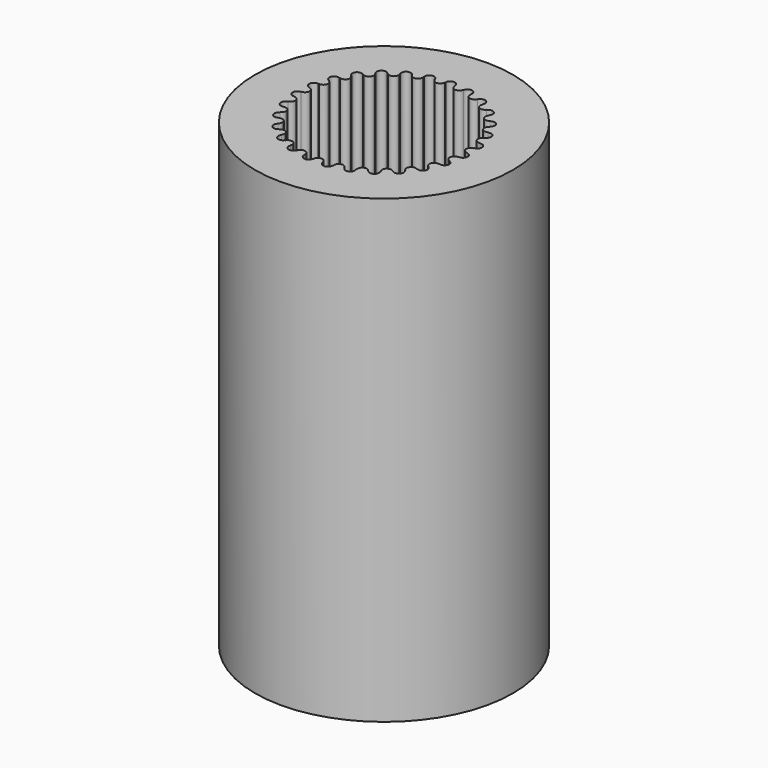
from build123d import *

# Parameters (mm, degrees)
F0_R     = 7
F1_DEPTH = 25


with BuildPart() as f1:
    # F0 (on Top) → F1 (new body)
    with BuildSketch(Plane.XY):
        Circle(F0_R)
        with BuildLine():
            ThreePointArc((4.4999467421, 0.0218933428), (4.4999866855, 0.0109467038), (4.5, 0))
            ThreePointArc((4.5, 0), (4.499999901, -0.0009440021), (4.4999996039, -0.0018880042))
            ThreePointArc((4.4999996039, -0.0018880042), (4.6722019825, -0.0775220264), (4.7429503115, -0.2517885994))
            ThreePointArc((4.7429503115, -0.2517885994), (4.6621704259, -0.4358118394), (4.4720338884, -0.5009120693))
            ThreePointArc((4.4720338884, -0.5009120693), (4.4706946769, -0.5127271263), (4.4693242502, -0.5245386035))
            ThreePointArc((4.4693242502, -0.5245386035), (4.6223829499, -0.6083851155), (4.6832973562, -0.7719291104))
            ThreePointArc((4.6832973562, -0.7719291104), (4.5915258656, -0.9654846291), (4.3835874457, -1.01693712))
            ThreePointArc((4.3835874457, -1.01693712), (4.3808850095, -1.0285166667), (4.3781519852, -1.040089032))
            ThreePointArc((4.3781519852, -1.040089032), (4.5119142579, -1.1293532515), (4.5636351508, -1.2816207651))
            ThreePointArc((4.5636351508, -1.2816207651), (4.460336155, -1.484053014), (4.2358046277, -1.5191968785))
            ThreePointArc((4.2358046277, -1.5191968785), (4.2317755471, -1.5303841736), (4.2277169195, -1.5415607832))
            ThreePointArc((4.2277169195, -1.5415607832), (4.3423845204, -1.6334890402), (4.3855834466, -1.7739643615))
            ThreePointArc((4.3855834466, -1.7739643615), (4.2702600875, -1.9845877277), (4.0306858273, -2.0008927411))
            ThreePointArc((4.0306858273, -2.0008927411), (4.0253846401, -2.011536353), (4.0200553469, -2.02216592))
            ThreePointArc((4.0200553469, -2.02216592), (4.116174988, -2.1140881649), (4.151552357, -2.2422955214))
            ThreePointArc((4.151552357, -2.2422955214), (4.0237485016, -2.4603966499), (3.7710075389, -2.4555044576))
            ThreePointArc((3.7710075389, -2.4555044576), (3.764506002, -2.4654603141), (3.7579781807, -2.4753989564))
            ThreePointArc((3.7579781807, -2.4753989564), (3.8364270221, -2.5647697304), (3.864709734, -2.6802748998))
            ThreePointArc((3.864709734, -2.6802748998), (3.7240115191, -2.9051151092), (3.4602847759, -2.8768783898))
            ThreePointArc((3.4602847759, -2.8768783898), (3.4526708943, -2.8860117282), (3.4450329057, -2.8951249159))
            ThreePointArc((3.4450329057, -2.8951249159), (3.5069993046, -2.9795622136), (3.5289382883, -3.0819739943))
            ThreePointArc((3.5289382883, -3.0819739943), (3.3749755225, -3.3127917788), (3.102723491, -3.2593108072))
            ThreePointArc((3.102723491, -3.2593108072), (3.0941003266, -3.2674979983), (3.0854555587, -3.2756623751))
            ThreePointArc((3.0854555587, -3.2756623751), (3.1324153628, -3.3529838574), (3.1487830325, -3.4419553935))
            ThreePointArc((3.1487830325, -3.4419553935), (2.9812304495, -3.677969002), (2.7031636451, -3.5976250927))
            ThreePointArc((2.7031636451, -3.5976250927), (2.6936479212, -3.6047553144), (2.6841133898, -3.611860367))
            ThreePointArc((2.6841133898, -3.611860367), (2.7178021206, -3.6801164221), (2.7293897599, -3.755346378))
            ThreePointArc((2.7293897599, -3.755346378), (2.5479681207, -3.9957564618), (2.2670136924, -3.8872418137))
            ThreePointArc((2.2670136924, -3.8872418137), (2.2567342142, -3.8932185511), (2.2464389791, -3.8991681053))
            ThreePointArc((2.2464389791, -3.8991681053), (2.268820309, -3.9566712966), (2.2764353908, -4.0179048778))
            ThreePointArc((2.2764353908, -4.0179048778), (2.080912429, -4.261897198), (1.8001773723, -4.1242407093))
            ThreePointArc((1.8001773723, -4.1242407093), (1.7892732831, -4.128983061), (1.7783567009, -4.1336965835))
            ThreePointArc((1.7783567009, -4.1336965835), (1.7915876777, -4.1790470769), (1.7960511297, -4.2260768929))
            ThreePointArc((1.7960511297, -4.2260768929), (1.5862423383, -4.4728250778), (1.3089737957, -4.3054137551))
            ThreePointArc((1.3089737957, -4.3054137551), (1.2975926935, -4.3088575286), (1.2862025314, -4.3122712169))
            ThreePointArc((1.2862025314, -4.3122712169), (1.2925960487, -4.3443778338), (1.2947394726, -4.3770446005))
            ThreePointArc((1.2947394726, -4.3770446005), (1.070508729, -4.6257129447), (0.8000519092, -4.4283085871))
            ThreePointArc((0.8000519092, -4.4283085871), (0.7883478491, -4.4304071674), (0.7766382847, -4.4324748138))
            ThreePointArc((0.7766382847, -4.4324748138), (0.7786233347, -4.4505714179), (0.7792861897, -4.468764497))
            ThreePointArc((0.7792861897, -4.468764497), (0.5405462167, -4.7185107918), (0.2803004953, -4.4912616972))
            ThreePointArc((0.2803004953, -4.4912616972), (0.2684319038, -4.4919866777), (0.2565614381, -4.4926802945))
            ThreePointArc((0.2565614381, -4.4926802945), (0.2566417125, -4.4963372852), (0.2566684725, -4.499995059))
            ThreePointArc((0.2566684725, -4.499995059), (0.0033811338, -4.7499734449), (-0.2432450747, -4.49342095))
            ThreePointArc((-0.2432450747, -4.49342095), (-0.255117544, -4.4927625175), (-0.2669882321, -4.4920727158))
            ThreePointArc((-0.2669882321, -4.4920727158), (-0.5447083709, -4.7186643015), (-0.7634980719, -4.4347571178))
            ThreePointArc((-0.7634980719, -4.4347571178), (-0.7752137129, -4.4327241849), (-0.7869239413, -4.4306603019))
            ThreePointArc((-0.7869239413, -4.4306603019), (-1.0890824956, -4.6234618326), (-1.2734163355, -4.3160642762))
            ThreePointArc((-1.2734163355, -4.3160642762), (-1.284816565, -4.3126843606), (-1.2962078237, -4.3092743331))
            ThreePointArc((-1.2962078237, -4.3092743331), (-1.618714766, -4.4656760413), (-1.7660975963, -4.1389490551))
            ThreePointArc((-1.7660975963, -4.1389490551), (-1.7770281003, -4.1342679075), (-1.7879461969, -4.1295578937))
            ThreePointArc((-1.7879461969, -4.1295578937), (-2.1264360633, -4.2474427211), (-2.2348729054, -3.9058088915))
            ThreePointArc((-2.2348729054, -3.9058088915), (-2.2451857283, -3.899889876), (-2.255482875, -3.8939436309))
            ThreePointArc((-2.255482875, -3.8939436309), (-2.6053738563, -3.9717158847), (-2.6733969057, -3.619799578))
            ThreePointArc((-2.6733969057, -3.619799578), (-2.6829524529, -3.6127228147), (-2.6924892672, -3.6056208267))
            ThreePointArc((-2.6924892672, -3.6056208267), (-3.0490452281, -3.6422277794), (-3.0757337228, -3.2847925454))
            ThreePointArc((-3.0757337228, -3.2847925454), (-3.0844026501, -3.2766538255), (-3.0930500415, -3.2684922274))
            ThreePointArc((-3.0930500415, -3.2684922274), (-3.4514446295, -3.2634383661), (-3.4364373131, -2.9053224594))
            ThreePointArc((-3.4364373131, -2.9053224594), (-3.4441022776, -2.8962319489), (-3.4517431947, -2.8871212163))
            ThreePointArc((-3.4517431947, -2.8871212163), (-3.8071251696, -2.8404749503), (-3.7506251817, -2.4865258387))
            ThreePointArc((-3.7506251817, -2.4865258387), (-3.7571824301, -2.476606587), (-3.7637134453, -2.4666700432))
            ThreePointArc((-3.7637134453, -2.4666700432), (-4.1112723457, -2.3790627776), (-4.0140444718, -2.0340715273))
            ThreePointArc((-4.0140444718, -2.0340715273), (-4.0194052451, -2.0234578017), (-4.0247379543, -2.012829948))
            ThreePointArc((-4.0247379543, -2.012829948), (-4.3597692121, -1.8854475376), (-4.2231295318, -1.5540839609))
            ThreePointArc((-4.2231295318, -1.5540839609), (-4.2272212664, -1.5429194291), (-4.2312834858, -1.5317441244))
            ThreePointArc((-4.2312834858, -1.5317441244), (-4.5492521077, -1.3663108214), (-4.3750501799, -1.0530602659))
            ThreePointArc((-4.3750501799, -1.0530602659), (-4.3778174899, -1.0414960514), (-4.3805542332, -1.029924565))
            ThreePointArc((-4.3805542332, -1.029924565), (-4.677156186, -0.8286796797), (-4.4677500134, -0.5377823145))
            ThreePointArc((-4.4677500134, -0.5377823145), (-4.4691554405, -0.5259749509), (-4.4705296631, -0.5141639148))
            ThreePointArc((-4.4705296631, -0.5141639148), (-4.7417501336, -0.2798315043), (-4.4999742446, -0.0152249251))
            ThreePointArc((-4.4999742446, -0.0152249251), (-4.4999987648, -0.0033342372), (-4.4999918652, 0.0085564741))
            ThreePointArc((-4.4999918652, 0.0085564741), (-4.7421596047, 0.2728044791), (-4.4712866852, 0.5075385493))
            ThreePointArc((-4.4712866852, 0.5075385493), (-4.4699299666, 0.5193516089), (-4.4685420382, 0.5311610422))
            ThreePointArc((-4.4685420382, 0.5311610422), (-4.6783790567, 0.8217477726), (-4.3820756509, 1.0234319662))
            ThreePointArc((-4.3820756509, 1.0234319662), (-4.3793560582, 1.0350074955), (-4.376605888, 1.0465757981))
            ThreePointArc((-4.376605888, 1.0465757981), (-4.5512718251, 1.3595678629), (-4.2335487052, 1.5254721764))
            ThreePointArc((-4.2335487052, 1.5254721764), (-4.2295030507, 1.5366534886), (-4.2254278651, 1.5478240716))
            ThreePointArc((-4.2254278651, 1.5478240716), (-4.3625584374, 1.8789848005), (-4.0277163132, 2.0068635481))
            ThreePointArc((-4.0277163132, 2.0068635481), (-4.0223993592, 2.0174992926), (-4.01705432, 2.0281209505))
            ThreePointArc((-4.01705432, 2.0281209505), (-4.1147933237, 2.3729677417), (-3.7673646286, 2.4610899526))
            ThreePointArc((-3.7673646286, 2.4610899526), (-3.7608483455, 2.4710361637), (-3.7543058034, 2.4809651216))
            ThreePointArc((-3.7543058034, 2.4809651216), (-3.8113302403, 2.8348301182), (-3.4560177799, 2.8820029675))
            ThreePointArc((-3.4560177799, 2.8820029675), (-3.4483903723, 2.891125013), (-3.4407388873, 2.9002268721))
            ThreePointArc((-3.4407388873, 2.9002268721), (-3.456276873, 3.2583201465), (-3.0978901677, 3.2639051011))
            ThreePointArc((-3.0978901677, 3.2639051011), (-3.0892548803, 3.2720795046), (-3.0805980232, 3.2802310619))
            ThreePointArc((-3.0805980232, 3.2802310619), (-3.054439235, 3.6377054526), (-2.6978294184, 3.6016269142))
            ThreePointArc((-2.6978294184, 3.6016269142), (-2.6883031388, 3.6087430269), (-2.678758089, 3.6158339426))
            ThreePointArc((-2.678758089, 3.6158339426), (-2.611256613, 3.9678506652), (-2.2612507666, 3.8905969941))
            ThreePointArc((-2.2612507666, 3.8905969941), (-2.2509624428, 3.8965584919), (-2.2406584025, 3.9024927833))
            ThreePointArc((-2.2406584025, 3.9024927833), (-2.1327279408, 4.2442869284), (-1.7940637545, 4.1269038328))
            ThreePointArc((-1.7940637545, 4.1269038328), (-1.7831526496, 4.1316300207), (-1.7722290945, 4.1363273609))
            ThreePointArc((-1.7722290945, 4.1363273609), (-1.6253305972, 4.4632723925), (-1.3025922399, 4.3073487735))
            ThreePointArc((-1.3025922399, 4.3073487735), (-1.291206047, 4.3107756778), (-1.2798108387, 4.3141724835))
            ThreePointArc((-1.2798108387, 4.3141724835), (-1.0959327283, 4.6218428635), (-0.7934887965, 4.429489308))
            ThreePointArc((-0.7934887965, 4.429489308), (-0.7817816394, 4.431570542), (-0.7700690238, 4.4336208339))
            ThreePointArc((-0.7700690238, 4.4336208339), (-0.5517002802, 4.7178519265), (-0.2736446642, 4.4916721383))
            ThreePointArc((-0.2736446642, 4.4916721383), (-0.2617750113, 4.4923795302), (-0.2499035308, 4.4930555556))
            ThreePointArc((-0.2499035308, 4.4930555556), (-0.0034725572, 4.7499758815), (0.25, 4.5))
            ThreePointArc((0.25, 4.5), (0.2499758815, 4.4965274428), (0.2499035308, 4.4930555556))
            ThreePointArc((0.2499035308, 4.4930555556), (0.255117544, 4.4927625175), (0.2603312137, 4.4924634288))
            ThreePointArc((0.2603312137, 4.4924634288), (0.5201193193, 4.7208440575), (0.759414462, 4.4710733505))
            ThreePointArc((0.759414462, 4.4710733505), (0.758791431, 4.4534345488), (0.7569254433, 4.4358836632))
            ThreePointArc((0.7569254433, 4.4358836632), (0.7686440841, 4.4338680937), (0.780357358, 4.4318215661))
            ThreePointArc((0.780357358, 4.4318215661), (1.0504868514, 4.6303708881), (1.2752704044, 4.3816458777))
            ThreePointArc((1.2752704044, 4.3816458777), (1.2731989807, 4.3495301331), (1.267019036, 4.317946591))
            ThreePointArc((1.267019036, 4.317946591), (1.2784242616, 4.3145835729), (1.289820561, 4.3111904296))
            ThreePointArc((1.289820561, 4.3111904296), (1.5668908867, 4.4797452241), (1.777248255, 4.2329083108))
            ThreePointArc((1.777248255, 4.2329083108), (1.7728887354, 4.1864243953), (1.7599622198, 4.1415616602))
            ThreePointArc((1.7599622198, 4.1415616602), (1.7708996487, 4.1368967154), (1.781824713, 4.1322028861))
            ThreePointArc((1.781824713, 4.1322028861), (2.0624877777, 4.2709867763), (2.2585532259, 4.0268739661))
            ThreePointArc((2.2585532259, 4.0268739661), (2.2510736567, 3.966179315), (2.2290825005, 3.9091164226))
            ThreePointArc((2.2290825005, 3.9091164226), (2.2394040835, 3.9032126961), (2.2497100305, 3.8972817166))
            ThreePointArc((2.2497100305, 3.8972817166), (2.5307141606, 4.0068936583), (2.7126703583, 3.7663317308))
            ThreePointArc((2.7126703583, 3.7663317308), (2.7012493529, 3.6916319093), (2.6680298516, 3.6237572643))
            ThreePointArc((2.6680298516, 3.6237572643), (2.6775958753, 3.616694669), (2.6871432035, 3.6096068212))
            ThreePointArc((2.6871432035, 3.6096068212), (2.9653753054, 3.6910046043), (3.1334527085, 3.4548083127))
            ThreePointArc((3.1334527085, 3.4548083127), (3.1172822297, 3.3663563198), (3.0708626682, 3.2893468156))
            ThreePointArc((3.0708626682, 3.2893468156), (3.0795436465, 3.281220951), (3.088203123, 3.2730721763))
            ThreePointArc((3.088203123, 3.2730721763), (3.3607284835, 3.3275511906), (3.5152045537, 3.0965205025))
            ThreePointArc((3.5152045537, 3.0965205025), (3.4934926499, 2.9946159141), (3.4321281926, 2.9104116667))
            ThreePointArc((3.4321281926, 2.9104116667), (3.4398066197, 2.9013325247), (3.4474610295, 2.8922331251))
            ThreePointArc((3.4474610295, 2.8922331251), (3.7115602241, 2.9214007075), (3.8527584891, 2.696318095))
            ThreePointArc((3.8527584891, 2.696318095), (3.824731977, 2.5813060492), (3.7469363237, 2.4920810954))
            ThreePointArc((3.7469363237, 2.4920810954), (3.7535082641, 2.4821715717), (3.7600539969, 2.472244717))
            ThreePointArc((3.7600539969, 2.472244717), (4.0132564165, 2.4779904525), (4.1415453741, 2.2596182423))
            ThreePointArc((4.1415453741, 2.2596182423), (4.1064524572, 2.1318882707), (4.0110258089, 2.0400176373))
            ThreePointArc((4.0110258089, 2.0400176373), (4.0164023046, 2.0294118674), (4.0217507571, 2.0187919278))
            ThreePointArc((4.0217507571, 2.0187919278), (4.2618643103, 2.0032543356), (4.3776561806, 1.7923321273))
            ThreePointArc((4.3776561806, 1.7923321273), (4.3347689953, 1.6523168353), (4.2208219246, 1.5603404375))
            ThreePointArc((4.2208219246, 1.5603404375), (4.2249301992, 1.5491819814), (4.2290089747, 1.5380127087))
            ThreePointArc((4.2290089747, 1.5380127087), (4.454145576, 1.5035427883), (4.5578949054, 1.3007849491))
            ThreePointArc((4.5578949054, 1.3007849491), (4.5065119864, 1.1489585511), (4.3734848642, 1.0595424212))
            ThreePointArc((4.3734848642, 1.0595424212), (4.376269308, 1.0479823202), (4.379023196, 1.036414902))
            ThreePointArc((4.379023196, 1.036414902), (4.5876197103, 0.9855370602), (4.6798218315, 0.7916303057))
            ThreePointArc((4.6798218315, 0.7916303057), (4.6192704875, 0.6285070187), (4.4669481775, 0.5444024059))
            ThreePointArc((4.4669481775, 0.5444024059), (4.4683711002, 0.5325971379), (4.4697628239, 0.5207881512))
            ThreePointArc((4.4697628239, 0.5207881512), (4.6605971976, 0.4561590617), (4.7417865523, 0.2717601299))
            ThreePointArc((4.7417865523, 0.2717601299), (4.6714251443, 0.0978924323), (4.4999467421, 0.0218933428))
        make_face(mode=Mode.SUBTRACT)
        with BuildLine():
            ThreePointArc((4.4697628239, 0.5207881512), (4.4917865523, 0.2717601299), (4.4999467421, 0.0218933428))
            ThreePointArc((4.4999467421, 0.0218933428), (4.6714251443, 0.0978924323), (4.7417865523, 0.2717601299))
            ThreePointArc((4.7417865523, 0.2717601299), (4.6605971976, 0.4561590617), (4.4697628239, 0.5207881512))
        make_face()
        with BuildLine():
            ThreePointArc((4.6832973562, -0.7719291104), (4.6223829499, -0.6083851155), (4.4693242502, -0.5245386035))
            ThreePointArc((4.4693242502, -0.5245386035), (4.4332973562, -0.7719291104), (4.3835874457, -1.01693712))
            ThreePointArc((4.3835874457, -1.01693712), (4.5915258656, -0.9654846291), (4.6832973562, -0.7719291104))
        make_face()
        with BuildLine():
            ThreePointArc((4.2290089747, 1.5380127087), (4.3078949054, 1.3007849491), (4.3734848642, 1.0595424212))
            ThreePointArc((4.3734848642, 1.0595424212), (4.5065119864, 1.1489585511), (4.5578949054, 1.3007849491))
            ThreePointArc((4.5578949054, 1.3007849491), (4.454145576, 1.5035427883), (4.2290089747, 1.5380127087))
        make_face()
        with BuildLine():
            ThreePointArc((4.3855834466, -1.7739643615), (4.3423845204, -1.6334890402), (4.2277169195, -1.5415607832))
            ThreePointArc((4.2277169195, -1.5415607832), (4.1355834466, -1.7739643615), (4.0306858273, -2.0008927411))
            ThreePointArc((4.0306858273, -2.0008927411), (4.2702600875, -1.9845877277), (4.3855834466, -1.7739643615))
        make_face()
        with BuildLine():
            ThreePointArc((3.7600539969, 2.472244717), (3.8915453741, 2.2596182423), (4.0110258089, 2.0400176373))
            ThreePointArc((4.0110258089, 2.0400176373), (4.1064524572, 2.1318882707), (4.1415453741, 2.2596182423))
            ThreePointArc((4.1415453741, 2.2596182423), (4.0132564165, 2.4779904525), (3.7600539969, 2.472244717))
        make_face()
        with BuildLine():
            ThreePointArc((3.864709734, -2.6802748998), (3.8364270221, -2.5647697304), (3.7579781807, -2.4753989564))
            ThreePointArc((3.7579781807, -2.4753989564), (3.614709734, -2.6802748998), (3.4602847759, -2.8768783898))
            ThreePointArc((3.4602847759, -2.8768783898), (3.7240115191, -2.9051151092), (3.864709734, -2.6802748998))
        make_face()
        with BuildLine():
            ThreePointArc((3.088203123, 3.2730721763), (3.2652045537, 3.0965205025), (3.4321281926, 2.9104116667))
            ThreePointArc((3.4321281926, 2.9104116667), (3.4934926499, 2.9946159141), (3.5152045537, 3.0965205025))
            ThreePointArc((3.5152045537, 3.0965205025), (3.3607284835, 3.3275511906), (3.088203123, 3.2730721763))
        make_face()
        with BuildLine():
            ThreePointArc((3.1487830325, -3.4419553935), (3.1324153628, -3.3529838574), (3.0854555587, -3.2756623751))
            ThreePointArc((3.0854555587, -3.2756623751), (2.8987830325, -3.4419553935), (2.7031636451, -3.5976250927))
            ThreePointArc((2.7031636451, -3.5976250927), (2.9812304495, -3.677969002), (3.1487830325, -3.4419553935))
        make_face()
        with BuildLine():
            ThreePointArc((2.2497100305, 3.8972817166), (2.4626703583, 3.7663317308), (2.6680298516, 3.6237572643))
            ThreePointArc((2.6680298516, 3.6237572643), (2.7012493529, 3.6916319093), (2.7126703583, 3.7663317308))
            ThreePointArc((2.7126703583, 3.7663317308), (2.5307141606, 4.0068936583), (2.2497100305, 3.8972817166))
        make_face()
        with BuildLine():
            ThreePointArc((2.2764353908, -4.0179048778), (2.268820309, -3.9566712966), (2.2464389791, -3.8991681053))
            ThreePointArc((2.2464389791, -3.8991681053), (2.0264353908, -4.0179048778), (1.8001773723, -4.1242407093))
            ThreePointArc((1.8001773723, -4.1242407093), (2.080912429, -4.261897198), (2.2764353908, -4.0179048778))
        make_face()
        with BuildLine():
            ThreePointArc((1.289820561, 4.3111904296), (1.527248255, 4.2329083108), (1.7599622198, 4.1415616602))
            ThreePointArc((1.7599622198, 4.1415616602), (1.7728887354, 4.1864243953), (1.777248255, 4.2329083108))
            ThreePointArc((1.777248255, 4.2329083108), (1.5668908867, 4.4797452241), (1.289820561, 4.3111904296))
        make_face()
        with BuildLine():
            ThreePointArc((1.2947394726, -4.3770446005), (1.2925960487, -4.3443778338), (1.2862025314, -4.3122712169))
            ThreePointArc((1.2862025314, -4.3122712169), (1.0447394726, -4.3770446005), (0.8000519092, -4.4283085871))
            ThreePointArc((0.8000519092, -4.4283085871), (1.070508729, -4.6257129447), (1.2947394726, -4.3770446005))
        make_face()
        with BuildLine():
            ThreePointArc((0.2603312137, 4.4924634288), (0.509414462, 4.4710733505), (0.7569254433, 4.4358836632))
            ThreePointArc((0.7569254433, 4.4358836632), (0.758791431, 4.4534345488), (0.759414462, 4.4710733505))
            ThreePointArc((0.759414462, 4.4710733505), (0.5201193193, 4.7208440575), (0.2603312137, 4.4924634288))
        make_face()
        with BuildLine():
            ThreePointArc((0.2566684725, -4.499995059), (0.2566417125, -4.4963372852), (0.2565614381, -4.4926802945))
            ThreePointArc((0.2565614381, -4.4926802945), (0.0066684725, -4.499995059), (-0.2432450747, -4.49342095))
            ThreePointArc((-0.2432450747, -4.49342095), (0.0033811338, -4.7499734449), (0.2566684725, -4.499995059))
        make_face()
        with BuildLine():
            ThreePointArc((-0.7700690238, 4.4336208339), (-0.5226634233, 4.4695439304), (-0.2736446642, 4.4916721383))
            ThreePointArc((-0.2736446642, 4.4916721383), (-0.5517002802, 4.7178519265), (-0.7700690238, 4.4336208339))
        make_face()
        with BuildLine():
            ThreePointArc((-1.2734163355, -4.3160642762), (-1.0890824956, -4.6234618326), (-0.7869239413, -4.4306603019))
            ThreePointArc((-0.7869239413, -4.4306603019), (-1.0317623643, -4.3801217362), (-1.2734163355, -4.3160642762))
        make_face()
        with BuildLine():
            ThreePointArc((-1.7722290945, 4.1363273609), (-1.5397868815, 4.2283633192), (-1.3025922399, 4.3073487735))
            ThreePointArc((-1.3025922399, 4.3073487735), (-1.6253305972, 4.4632723925), (-1.7722290945, 4.1363273609))
        make_face()
        with BuildLine():
            ThreePointArc((-2.2348729054, -3.9058088915), (-2.1264360633, -4.2474427211), (-1.7879461969, -4.1295578937))
            ThreePointArc((-1.7879461969, -4.1295578937), (-2.0145183758, -4.0238931042), (-2.2348729054, -3.9058088915))
        make_face()
        with BuildLine():
            ThreePointArc((-2.678758089, 3.6158339426), (-2.4738220544, 3.7590164196), (-2.2612507666, 3.8905969941))
            ThreePointArc((-2.2612507666, 3.8905969941), (-2.611256613, 3.9678506652), (-2.678758089, 3.6158339426))
        make_face()
        with BuildLine():
            ThreePointArc((-3.0757337228, -3.2847925454), (-3.0490452281, -3.6422277794), (-2.6924892672, -3.6056208267))
            ThreePointArc((-2.6924892672, -3.6056208267), (-2.8885691635, -3.4505315805), (-3.0757337228, -3.2847925454))
        make_face()
        with BuildLine():
            ThreePointArc((-3.4407388873, 2.9002268721), (-3.2743675639, 3.0868296125), (-3.0978901677, 3.2639051011))
            ThreePointArc((-3.0978901677, 3.2639051011), (-3.456276873, 3.2583201465), (-3.4407388873, 2.9002268721))
        make_face()
        with BuildLine():
            ThreePointArc((-3.7506251817, -2.4865258387), (-3.8071251696, -2.8404749503), (-3.4517431947, -2.8871212163))
            ThreePointArc((-3.4517431947, -2.8871212163), (-3.6067501607, -2.6909762687), (-3.7506251817, -2.4865258387))
        make_face()
        with BuildLine():
            ThreePointArc((-4.01705432, 2.0281209505), (-3.898225254, 2.2480747027), (-3.7673646286, 2.4610899526))
            ThreePointArc((-3.7673646286, 2.4610899526), (-4.1147933237, 2.3729677417), (-4.01705432, 2.0281209505))
        make_face()
        with BuildLine():
            ThreePointArc((-4.2231295318, -1.5540839609), (-4.3597692121, -1.8854475376), (-4.0247379543, -2.012829948))
            ThreePointArc((-4.0247379543, -2.012829948), (-4.1303076746, -1.7862134567), (-4.2231295318, -1.5540839609))
        make_face()
        with BuildLine():
            ThreePointArc((-4.376605888, 1.0465757981), (-4.3117312028, 1.2880116596), (-4.2335487052, 1.5254721764))
            ThreePointArc((-4.2335487052, 1.5254721764), (-4.5512718251, 1.3595678629), (-4.376605888, 1.0465757981))
        make_face()
        with BuildLine():
            ThreePointArc((-4.4677500134, -0.5377823145), (-4.677156186, -0.8286796797), (-4.3805542332, -1.029924565))
            ThreePointArc((-4.3805542332, -1.029924565), (-4.430990071, -0.7850649598), (-4.4677500134, -0.5377823145))
        make_face()
        with BuildLine():
            ThreePointArc((-4.4999918652, 0.0085564741), (-4.4925722571, 0.2584463486), (-4.4712866852, 0.5075385493))
            ThreePointArc((-4.4712866852, 0.5075385493), (-4.7421596047, 0.2728044791), (-4.4999918652, 0.0085564741))
        make_face()
        with BuildLine():
            ThreePointArc((4.4697628239, 0.5207881512), (4.242242855, 0.2566623449), (4.4999467421, 0.0218933428))
            ThreePointArc((4.4999467421, 0.0218933428), (4.4917865523, 0.2717601299), (4.4697628239, 0.5207881512))
        make_face()
        with BuildLine():
            ThreePointArc((4.3835874457, -1.01693712), (4.4332973562, -0.7719291104), (4.4693242502, -0.5245386035))
            ThreePointArc((4.4693242502, -0.5245386035), (4.1870030586, -0.7290441598), (4.3835874457, -1.01693712))
        make_face()
        with BuildLine():
            ThreePointArc((4.2290089747, 1.5380127087), (4.0685674107, 1.2285191186), (4.3734848642, 1.0595424212))
            ThreePointArc((4.3734848642, 1.0595424212), (4.3078949054, 1.3007849491), (4.2290089747, 1.5380127087))
        make_face()
        with BuildLine():
            ThreePointArc((4.0306858273, -2.0008927411), (4.1355834466, -1.7739643615), (4.2277169195, -1.5415607832))
            ThreePointArc((4.2277169195, -1.5415607832), (3.9058288107, -1.6754107858), (4.0306858273, -2.0008927411))
        make_face()
        with BuildLine():
            ThreePointArc((3.7600539969, 2.472244717), (3.6753484089, 2.1340838955), (4.0110258089, 2.0400176373))
            ThreePointArc((4.0110258089, 2.0400176373), (3.8915453741, 2.2596182423), (3.7600539969, 2.472244717))
        make_face()
        with BuildLine():
            ThreePointArc((3.4602847759, -2.8768783898), (3.614709734, -2.6802748998), (3.7579781807, -2.4753989564))
            ThreePointArc((3.7579781807, -2.4753989564), (3.4138925266, -2.5313707387), (3.4602847759, -2.8768783898))
        make_face()
        with BuildLine():
            ThreePointArc((3.088203123, 3.2730721763), (3.0838043007, 2.9244915857), (3.4321281926, 2.9104116667))
            ThreePointArc((3.4321281926, 2.9104116667), (3.2652045537, 3.0965205025), (3.088203123, 3.2730721763))
        make_face()
        with BuildLine():
            ThreePointArc((2.7031636451, -3.5976250927), (2.8987830325, -3.4419553935), (3.0854555587, -3.2756623751))
            ThreePointArc((3.0854555587, -3.2756623751), (2.7377395307, -3.2507356494), (2.7031636451, -3.5976250927))
        make_face()
        with BuildLine():
            ThreePointArc((2.2497100305, 3.8972817166), (2.3258553384, 3.5570910791), (2.6680298516, 3.6237572643))
            ThreePointArc((2.6680298516, 3.6237572643), (2.4626703583, 3.7663317308), (2.2497100305, 3.8972817166))
        make_face()
        with BuildLine():
            ThreePointArc((1.8001773723, -4.1242407093), (2.0264353908, -4.0179048778), (2.2464389791, -3.8991681053))
            ThreePointArc((2.2464389791, -3.8991681053), (1.9138556469, -3.7946879401), (1.8001773723, -4.1242407093))
        make_face()
        with BuildLine():
            ThreePointArc((1.289820561, 4.3111904296), (1.4424011297, 3.997746738), (1.7599622198, 4.1415616602))
            ThreePointArc((1.7599622198, 4.1415616602), (1.527248255, 4.2329083108), (1.289820561, 4.3111904296))
        make_face()
        with BuildLine():
            ThreePointArc((0.8000519092, -4.4283085871), (1.0447394726, -4.3770446005), (1.2862025314, -4.3122712169))
            ThreePointArc((1.2862025314, -4.3122712169), (0.9866983908, -4.133875456), (0.8000519092, -4.4283085871))
        make_face()
        with BuildLine():
            ThreePointArc((0.2603312137, 4.4924634288), (0.4811136585, 4.2226803866), (0.7569254433, 4.4358836632))
            ThreePointArc((0.7569254433, 4.4358836632), (0.509414462, 4.4710733505), (0.2603312137, 4.4924634288))
        make_face()
        with BuildLine():
            ThreePointArc((-0.2432450747, -4.49342095), (0.0066684725, -4.499995059), (0.2565614381, -4.4926802945))
            ThreePointArc((0.2565614381, -4.4926802945), (0.0062980018, -4.2499953335), (-0.2432450747, -4.49342095))
        make_face()
        with BuildLine():
            ThreePointArc((-0.2726634233, 4.4695439304), (-0.272908854, 4.4806189069), (-0.2736446642, 4.4916721383))
            ThreePointArc((-0.2736446642, 4.4916721383), (-0.5226634233, 4.4695439304), (-0.7700690238, 4.4336208339))
            ThreePointArc((-0.7700690238, 4.4336208339), (-0.5046550935, 4.2201933739), (-0.2726634233, 4.4695439304))
        make_face()
        with BuildLine():
            ThreePointArc((-1.2734163355, -4.3160642762), (-1.0317623643, -4.3801217362), (-0.7869239413, -4.4306603019))
            ThreePointArc((-0.7869239413, -4.4306603019), (-0.7830561061, -4.405522467), (-0.7817623643, -4.3801217362))
            ThreePointArc((-0.7817623643, -4.3801217362), (-0.9994629279, -4.1322170238), (-1.2734163355, -4.3160642762))
        make_face()
        with BuildLine():
            ThreePointArc((-1.2897868815, 4.2283633192), (-1.293008985, 4.2683716908), (-1.3025922399, 4.3073487735))
            ThreePointArc((-1.3025922399, 4.3073487735), (-1.5397868815, 4.2283633192), (-1.7722290945, 4.1363273609))
            ThreePointArc((-1.7722290945, 4.1363273609), (-1.4929390067, 3.9827919923), (-1.2897868815, 4.2283633192))
        make_face()
        with BuildLine():
            ThreePointArc((-2.2348729054, -3.9058088915), (-2.0145183758, -4.0238931042), (-1.7879461969, -4.1295578937))
            ThreePointArc((-1.7879461969, -4.1295578937), (-1.7704455949, -4.0780085145), (-1.7645183758, -4.0238931042))
            ThreePointArc((-1.7645183758, -4.0238931042), (-1.9536440478, -3.7814177112), (-2.2348729054, -3.9058088915))
        make_face()
        with BuildLine():
            ThreePointArc((-2.2238220544, 3.7590164196), (-2.233361224, 3.8274166318), (-2.2612507666, 3.8905969941))
            ThreePointArc((-2.2612507666, 3.8905969941), (-2.4738220544, 3.7590164196), (-2.678758089, 3.6158339426))
            ThreePointArc((-2.678758089, 3.6158339426), (-2.3987687688, 3.5205483834), (-2.2238220544, 3.7590164196))
        make_face()
        with BuildLine():
            ThreePointArc((-3.0757337228, -3.2847925454), (-2.8885691635, -3.4505315805), (-2.6924892672, -3.6056208267))
            ThreePointArc((-2.6924892672, -3.6056208267), (-2.6524336367, -3.5326291625), (-2.6385691635, -3.4505315805))
            ThreePointArc((-2.6385691635, -3.4505315805), (-2.7999439409, -3.2167676613), (-3.0757337228, -3.2847925454))
        make_face()
        with BuildLine():
            ThreePointArc((-3.0243675639, 3.0868296125), (-3.0434786847, 3.1826957978), (-3.0978901677, 3.2639051011))
            ThreePointArc((-3.0978901677, 3.2639051011), (-3.2743675639, 3.0868296125), (-3.4407388873, 2.9002268721))
            ThreePointArc((-3.4407388873, 2.9002268721), (-3.1721247912, 2.8586927776), (-3.0243675639, 3.0868296125))
        make_face()
        with BuildLine():
            ThreePointArc((-3.7506251817, -2.4865258387), (-3.6067501607, -2.6909762687), (-3.4517431947, -2.8871212163))
            ThreePointArc((-3.4517431947, -2.8871212163), (-3.3817482257, -2.7999447469), (-3.3567501607, -2.6909762687))
            ThreePointArc((-3.3567501607, -2.6909762687), (-3.4915736771, -2.4690880589), (-3.7506251817, -2.4865258387))
        make_face()
        with BuildLine():
            ThreePointArc((-3.648225254, 2.2480747027), (-3.6800336452, 2.3701092135), (-3.7673646286, 2.4610899526))
            ThreePointArc((-3.7673646286, 2.4610899526), (-3.898225254, 2.2480747027), (-4.01705432, 2.0281209505))
            ThreePointArc((-4.01705432, 2.0281209505), (-3.7701769555, 2.0333571364), (-3.648225254, 2.2480747027))
        make_face()
        with BuildLine():
            ThreePointArc((-4.2231295318, -1.5540839609), (-4.1303076746, -1.7862134567), (-4.0247379543, -2.012829948))
            ThreePointArc((-4.0247379543, -2.012829948), (-3.9194849646, -1.9205778305), (-3.8803076746, -1.7862134567))
            ThreePointArc((-3.8803076746, -1.7862134567), (-3.9901389625, -1.579204442), (-4.2231295318, -1.5540839609))
        make_face()
        with BuildLine():
            ThreePointArc((-4.0617312028, 1.2880116596), (-4.1091903126, 1.4345626329), (-4.2335487052, 1.5254721764))
            ThreePointArc((-4.2335487052, 1.5254721764), (-4.3117312028, 1.2880116596), (-4.376605888, 1.0465757981))
            ThreePointArc((-4.376605888, 1.0465757981), (-4.1596106442, 1.0896197856), (-4.0617312028, 1.2880116596))
        make_face()
        with BuildLine():
            ThreePointArc((-4.4677500134, -0.5377823145), (-4.430990071, -0.7850649598), (-4.3805542332, -1.029924565))
            ThreePointArc((-4.3805542332, -1.029924565), (-4.2372002887, -0.9430064688), (-4.180990071, -0.7850649598))
            ThreePointArc((-4.180990071, -0.7850649598), (-4.2677264584, -0.5957372206), (-4.4677500134, -0.5377823145))
        make_face()
        with BuildLine():
            ThreePointArc((-4.2425722571, 0.2584463486), (-4.3084236853, 0.4275300661), (-4.4712866852, 0.5075385493))
            ThreePointArc((-4.4712866852, 0.5075385493), (-4.4925722571, 0.2584463486), (-4.4999918652, 0.0085564741))
            ThreePointArc((-4.4999918652, 0.0085564741), (-4.318438547, 0.0790656055), (-4.2425722571, 0.2584463486))
        make_face()
    extrude(amount=F1_DEPTH)


solid = f1.part
